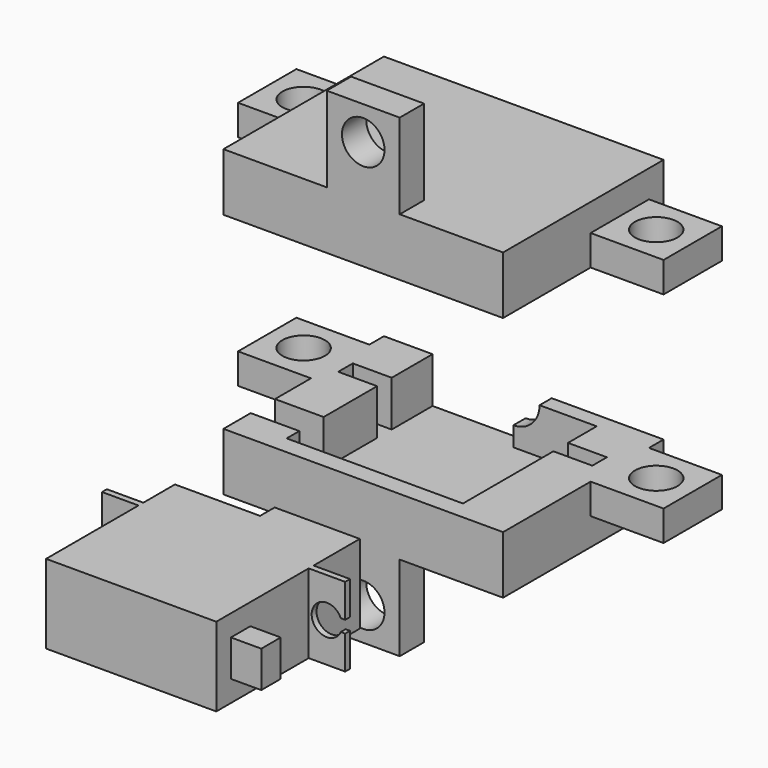
from build123d import *

# Parameters (mm, degrees)
F0_W      = 28
F0_H      = 29.5
F1_DEPTH  = 13
F3_DEPTH  = 3
F4_R      = 3
F4_R_2    = 1
F5_DEPTH  = 4
F6_W      = 1
F6_H      = 13
F7_DEPTH  = 6
F8_W      = 1
F8_H      = 13
F9_DEPTH  = 6
F11_DEPTH = 1
F13_DEPTH = 1
F14_W     = 4
F14_H     = 6
F15_DEPTH = 5
F16_W     = 12
F16_H     = 5
F17_DEPTH = 19
F19_W     = 29
F19_H     = 14
F20_DEPTH = 26.5
F21_W     = 33
F21_H     = 9.5
F22_DEPTH = 46
F24_DEPTH = 4
F25_W     = 6.4
F25_H     = 3
F26_DEPTH = 7.5
F27_W     = 9
F27_H     = 5
F28_DEPTH = 6.8
F31_W     = 12
F31_H     = 5
F32_DEPTH = 12
F33_W     = 12
F33_H     = 5
F34_DEPTH = 12
F35_R     = 3.5
F36_DEPTH = 5
F37_R     = 3.5
F38_DEPTH = 5
F39_DEPTH = 1
F40_DEPTH = 14
F41_R     = 3.5
F42_DEPTH = 5


# Not quite as in the source:
# - a feature names something its author has since deleted; it is built from what else it names


with BuildPart() as f1:
    # F0 (on Top) → F1 (new body)
    with BuildSketch(Plane.XY):
        Rectangle(F0_W, F0_H)
    extrude(amount=F1_DEPTH)

    # F2 (on face) → F3 (cut)
    with BuildSketch(Plane(origin=(0, 14.75, 0), x_dir=(-1, 0, 0), z_dir=(0, 1, 0))):
        with BuildLine():
            ThreePointArc((0, 10.5), (2.8284271247, 9.3284271247), (4, 6.5))
            ThreePointArc((4, 6.5), (2.8284271247, 3.6715728753), (0, 2.5))
            Line((0, 2.5), (0, 0))
            Line((0, 0), (14, 0))
            Line((14, 0), (14, 13))
            Line((14, 13), (0, 13))
            Line((0, 13), (0, 10.5))
        make_face()
    extrude(amount=-F3_DEPTH, mode=Mode.SUBTRACT)

    # F4 (on face) → F5 (join)
    with BuildSketch(Plane(origin=(0, 14.75, 0), x_dir=(-1, 0, 0), z_dir=(0, 1, 0))):
        with Locations((-7, 6.5)):
            Circle(F4_R)
        with Locations((-7, 6.5)):
            Circle(F4_R_2, mode=Mode.SUBTRACT)
    extrude(amount=F5_DEPTH)

    # F6 (on face) → F7 (join)
    with BuildSketch(Plane(origin=(-14, 0, 0), x_dir=(0, -1, 0), z_dir=(-1, 0, 0))):
        with Locations((-4.75, 6.5)):
            Rectangle(F6_W, F6_H)
    extrude(amount=F7_DEPTH)

    # F8 (on face) → F9 (join)
    with BuildSketch(Plane.YZ.offset(14)):
        with Locations((4.75, 6.5)):
            Rectangle(F8_W, F8_H)
    extrude(amount=F9_DEPTH)

    # F10 (on face) → F11 (cut)
    with BuildSketch(Plane(origin=(0, 5.25, 0), x_dir=(-1, 0, 0), z_dir=(0, 1, 0))):
        with BuildLine():
            Line((-20, 5.5), (-19.2775895342, 5.5))
            ThreePointArc((-19.2775895342, 5.5), (-14.4863016867, 6.5), (-19.2775895342, 7.5))
            Line((-19.2775895342, 7.5), (-20, 7.5))
            Line((-20, 7.5), (-20, 5.5))
        make_face()
    extrude(amount=-F11_DEPTH, mode=Mode.SUBTRACT)

    # F12 (on face) → F13 (cut)
    with BuildSketch(Plane(origin=(0, 5.25, 0), x_dir=(-1, 0, 0), z_dir=(0, 1, 0))):
        with BuildLine():
            Line((20, 7.5), (19.2912878475, 7.5))
            ThreePointArc((19.2912878475, 7.5), (14.5, 6.5), (19.2912878475, 5.5))
            Line((19.2912878475, 5.5), (20, 5.5))
            Line((20, 5.5), (20, 7.5))
        make_face()
    extrude(amount=-F13_DEPTH, mode=Mode.SUBTRACT)

    # F14 (on face) → F15 (join)
    with BuildSketch(Plane.YZ.offset(14)):
        with Locations((-9.75, 6.5)):
            Rectangle(F14_W, F14_H)
    extrude(amount=F15_DEPTH)


with BuildPart() as f17:
    # F16 (on Top) → F17 (new body)
    with BuildSketch(Plane.XY):
        Polygon((23, 65.9673700035), (-23, 65.9673700035), (-23, 32.9673700035), (-6, 32.9673700035), (-6, 37.9673700035), (6, 37.9673700035), (6, 32.9673700035), (23, 32.9673700035), align=None)
        with Locations((0, 35.4673700035)):
            Rectangle(F16_W, F16_H)
    extrude(amount=F17_DEPTH)

    # F19 (on offset) → F20 (cut)
    with BuildSketch(Plane.XZ.offset(-35.9673700035)):
        with Locations((-0.5, 9)):
            Rectangle(F19_W, F19_H)
    extrude(amount=-F20_DEPTH, mode=Mode.SUBTRACT)

    # F21 (on face) → F22 (cut)
    with BuildSketch(Plane(origin=(-23, 0, 0), x_dir=(0, -1, 0), z_dir=(-1, 0, 0))):
        with Locations((-49.4673700035, 14.25)):
            Rectangle(F21_W, F21_H)
    extrude(amount=-F22_DEPTH, mode=Mode.SUBTRACT)

    # F23 (on face) → F24 (cut)
    with BuildSketch(Plane(origin=(0, 65.9673700035, 0), x_dir=(-1, 0, 0), z_dir=(0, 1, 0))):
        with BuildLine():
            Line((4, 9.5), (-4.6, 9.5))
            ThreePointArc((-4.6, 9.5), (-3.3405591591, 6.4594408409), (-0.3, 5.2))
            Line((-0.3, 5.2), (-0.3, 2))
            Line((-0.3, 2), (15, 2))
            Line((15, 2), (15, 9.5))
            Line((15, 9.5), (4, 9.5))
        make_face()
    extrude(amount=-F24_DEPTH, mode=Mode.SUBTRACT)

    # F25 (on face) → F26 (cut)
    with BuildSketch(Plane.XY.offset(9.5)):
        with Locations((-18.2, 56.0673700035)):
            Rectangle(F25_W, F25_H)
        with Locations((17.2, 56.0673700035)):
            Rectangle(F25_W, F25_H)
    extrude(amount=-F26_DEPTH, mode=Mode.SUBTRACT)

    # F27 (on face) → F28 (cut)
    with BuildSketch(Plane.XY.offset(9.5)):
        with Locations((-19.5, 41.0718345642)):
            Rectangle(F27_W, F27_H)
    extrude(amount=-F28_DEPTH, mode=Mode.SUBTRACT)


with BuildPart() as f30_1:
    # F30: copy of F17
    add(f17.part)


with BuildPart() as f17_1:
    add(f17.part)

    add(f30_1.part)  # F32 merges F30_1
    # F31 (on face) → F32 (join)
    with BuildSketch(Plane.YZ.offset(23)):
        with Locations((56.9673700035, 7)):
            Rectangle(F31_W, F31_H)
    extrude(amount=F32_DEPTH)

    # F33 (on face) → F34 (join)
    with BuildSketch(Plane(origin=(-23, 0, 0), x_dir=(0, -1, 0), z_dir=(-1, 0, 0))):
        with Locations((-56.9673700035, 7)):
            Rectangle(F33_W, F33_H)
    extrude(amount=F34_DEPTH)

    # F35 (on face) → F36 (cut)
    with BuildSketch(Plane(origin=(0, 0, 4.5), x_dir=(1, 0, 0), z_dir=(0, 0, -1))):
        with Locations((-29, -56.9673700035)):
            Circle(F35_R)
    extrude(amount=-F36_DEPTH, mode=Mode.SUBTRACT)

    # F37 (on face) → F38 (cut)
    with BuildSketch(Plane(origin=(0, 0, 4.5), x_dir=(1, 0, 0), z_dir=(0, 0, -1))):
        with Locations((29, -56.9673700035)):
            Circle(F37_R)
    extrude(amount=-F38_DEPTH, mode=Mode.SUBTRACT)

    # F39 (cut): a face of the model
    f39_faces = [f17_1.faces().sort_by_distance(p)[0] for p in [
        (7.9771009102, 62.4673700035, 5.4331480297),
    ]]
    extrude(f39_faces, amount=-F39_DEPTH, mode=Mode.SUBTRACT)

    # F16 (on Top) → F40 (join)
    with BuildSketch(Plane.XY):
        with Locations((0, 35.4673700035)):
            Rectangle(F16_W, F16_H)
    extrude(amount=-F40_DEPTH)

    # F41 (on face) → F42 (cut)
    with BuildSketch(Plane.XZ.offset(-32.9673700035)):
        with Locations((0, -8.5)):
            Circle(F41_R)
    extrude(amount=-F42_DEPTH, mode=Mode.SUBTRACT)


with BuildPart() as f43_1:
    # F43: instance of F17
    add(f17_1.part.mirror(Plane.XY.offset(25)))


solid = Compound([f1.part, f17_1.part, f43_1.part])
